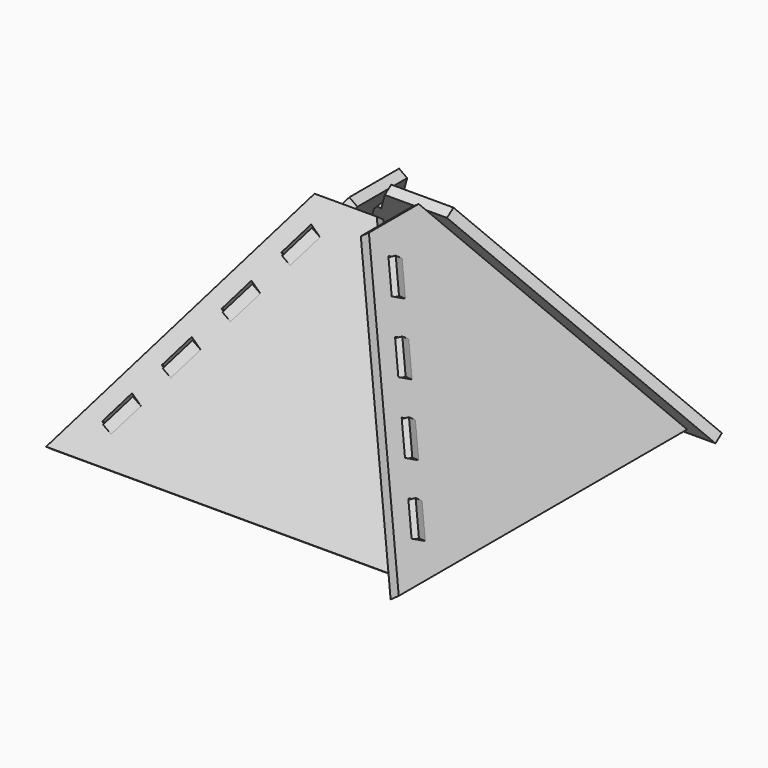
from build123d import *

# Parameters (mm, degrees)
F4_DEPTH = 3
F5_COUNT = 4


# Not quite as in the source:
# - a feature names something its author has since deleted; it is built from what else it names


with BuildPart() as f4:
    # F3 (on 3pt) → F4 (new body)
    with BuildSketch(Plane(origin=(33.3040282971, 0, 23.5805664487), x_dir=(0, -1, 0), z_dir=(-0.8161375901, 0, -0.5778576244))):
        Polygon((0, 48.9809723066), (0, -28.8928812192), (50, -28.8928812192), (60, -28.8928812192), (15, 48.9809723066), (5, 48.9809723066), align=None)
        Polygon((42.7786668474, -10.0351379853), (47.7819611302, -18.6934892325), (45.0263542623, -20.285837671), (44.1062312752, -20.8175377544), (39.1029369924, -12.1591865072), (40.0230599795, -11.6274864238), align=None, mode=Mode.SUBTRACT)
        Polygon((32.7720782819, 7.2815645091), (37.7753725646, -1.3767867381), (35.0197656967, -2.9691351766), (34.0996427097, -3.50083526), (29.0963484269, 5.1575159872), (30.0164714139, 5.6892160706), align=None, mode=Mode.SUBTRACT)
        Polygon((22.7654897163, 24.5982670035), (27.7687839991, 15.9399157563), (25.0131771311, 14.3475673178), (24.0930541441, 13.8158672344), (19.0897598613, 22.4742184816), (20.0098828484, 23.005918565), align=None, mode=Mode.SUBTRACT)
        Polygon((9.0831712957, 39.790920976), (10.0032942828, 40.3226210594), (12.7589011507, 41.9149694979), (17.7621954335, 33.2566182507), (15.0065885656, 31.6642698122), (14.0864655785, 31.1325697288), align=None, mode=Mode.SUBTRACT)
        Polygon((-48.7726300659, -28.8928812192), (0, -28.8928812192), (0, 48.9809723066), (-3.7726300659, 48.9809723066), (-9.0831712957, 39.790920976), (-10.0032942828, 40.3226210594), (-12.7589011507, 41.9149694979), (-17.7621954335, 33.2566182507), (-15.0065885656, 31.6642698122), (-14.0864655785, 31.1325697288), (-19.0897598613, 22.4742184816), (-20.0098828484, 23.005918565), (-22.7654897163, 24.5982670035), (-27.7687839991, 15.9399157563), (-25.0131771311, 14.3475673178), (-24.0930541441, 13.8158672344), (-29.0963484269, 5.1575159872), (-30.0164714139, 5.6892160706), (-32.7720782819, 7.2815645091), (-37.7753725646, -1.3767867381), (-35.0197656967, -2.9691351766), (-34.0996427097, -3.50083526), (-39.1029369924, -12.1591865072), (-40.0230599795, -11.6274864238), (-42.7786668474, -10.0351379853), (-47.7819611302, -18.6934892325), (-45.0263542623, -20.285837671), (-44.1062312752, -20.8175377544), align=None)
    extrude(amount=-F4_DEPTH)


with BuildPart() as f5_1:
    # F5: instance of F4
    add(f4.part.rotate(Axis((0, 0, 35.3087661927), (0, 0, -1)), 1 * 360 / F5_COUNT))


with BuildPart() as f5_2:
    # F5: instance of F4
    add(f4.part.rotate(Axis((0, 0, 35.3087661927), (0, 0, -1)), 2 * 360 / F5_COUNT))


with BuildPart() as f5_3:
    # F5: instance of F4
    add(f4.part.rotate(Axis((0, 0, 35.3087661927), (0, 0, -1)), 3 * 360 / F5_COUNT))


solid = Compound([f4.part, f5_1.part, f5_2.part, f5_3.part])
